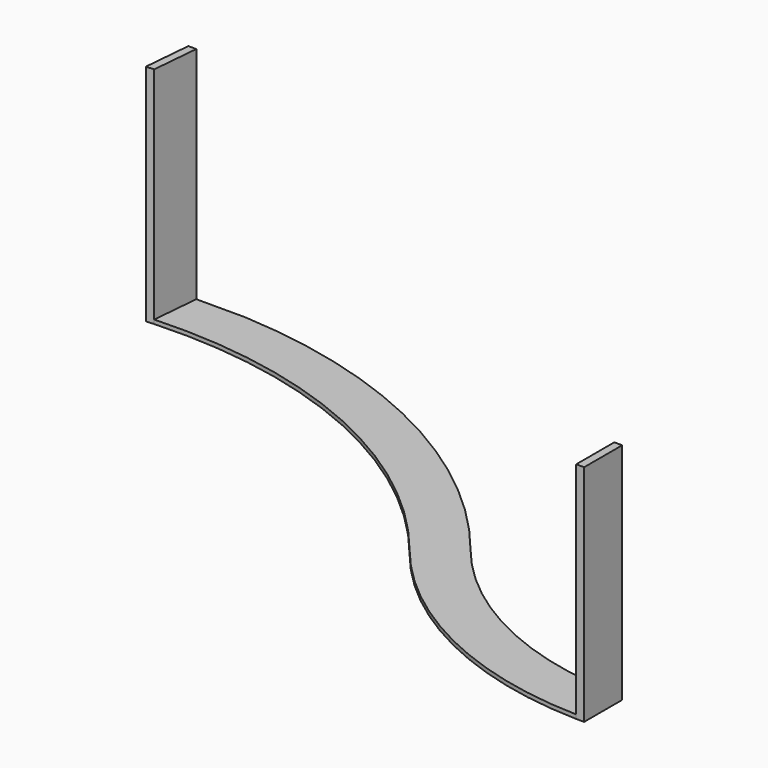
from build123d import *

# Parameters (mm, degrees)
F1_DEPTH = 25.4
F2_DEPTH = 1435.1
F3_DEPTH = 25.4
F4_DEPTH = 1435.1


with BuildPart() as f1:
    # F0 (on Top) → F1 (new body)
    with BuildSketch(Plane.XY):
        with BuildLine():
            Line((-1948.5691277788, 99.7355101007), (-2263.234400171, 99.7355101007))
            Line((-2263.234400171, 99.7355101007), (-2289.862411819, -203.7745007557))
            ThreePointArc((-2289.862411819, -203.7745007557), (-874.5398284023, -470.4550472357), (263.8832180742, -1352.6395496224))
            ThreePointArc((263.8832180742, -1352.6395496224), (346.7538874408, -1450.5053929427), (434.8963853674, -1543.651360055))
            Line((434.8963853674, -1543.651360055), (650.422532273, -1328.1252131493))
            ThreePointArc((650.422532273, -1328.1252131493), (573.8397062056, -1247.1951105763), (501.8373213462, -1162.1641319538))
            ThreePointArc((501.8373213462, -1162.1641319538), (-588.8138343544, -269.9358016898), (-1948.5691277788, 99.7355101007))
        make_face()
    extrude(amount=F1_DEPTH)

    # F0 (on Top) → F2 (join)
    with BuildSketch(Plane.XY):
        with BuildLine():
            Line((-2263.234400171, 99.7355101007), (-2314.2295336755, 99.7355101007))
            Line((-2314.2295336755, 99.7355101007), (-2341.1214825581, -206.7828963515))
            ThreePointArc((-2341.1214825581, -206.7828963515), (-2315.4982300933, -205.1716461899), (-2289.862411819, -203.7745007557))
            Line((-2289.862411819, -203.7745007557), (-2263.234400171, 99.7355101007))
        make_face()
    extrude(amount=F2_DEPTH)

    # F0 (on Top) → F3 (join)
    with BuildSketch(Plane.XY):
        with BuildLine():
            ThreePointArc((2027.483255523, -1918.925395054), (1282.1233486229, -1755.9858840328), (650.422532273, -1328.1252131493))
            Line((650.422532273, -1328.1252131493), (434.8963853674, -1543.651360055))
            ThreePointArc((434.8963853674, -1543.651360055), (1165.4738720531, -2037.6039199968), (2027.483255523, -2223.8092323134))
            Line((2027.483255523, -2223.8092323134), (2027.483255523, -1918.925395054))
        make_face()
    extrude(amount=F3_DEPTH)

    # F0 (on Top) → F4 (join)
    with BuildSketch(Plane.XY):
        with BuildLine():
            ThreePointArc((2052.883255523, -1919.4047351522), (2040.182501702, -1919.2050097162), (2027.483255523, -1918.925395054))
            Line((2027.483255523, -1918.925395054), (2027.483255523, -2223.8092323134))
            ThreePointArc((2027.483255523, -2223.8092323134), (2052.8817382899, -2224.225671357), (2078.283255523, -2224.3644898993))
            Line((2078.283255523, -2224.3644898993), (2078.283255523, -1919.5644898993))
            ThreePointArc((2078.283255523, -1919.5644898993), (2065.5830043289, -1919.5245508176), (2052.883255523, -1919.4047351522))
        make_face()
    extrude(amount=F4_DEPTH)


solid = f1.part
